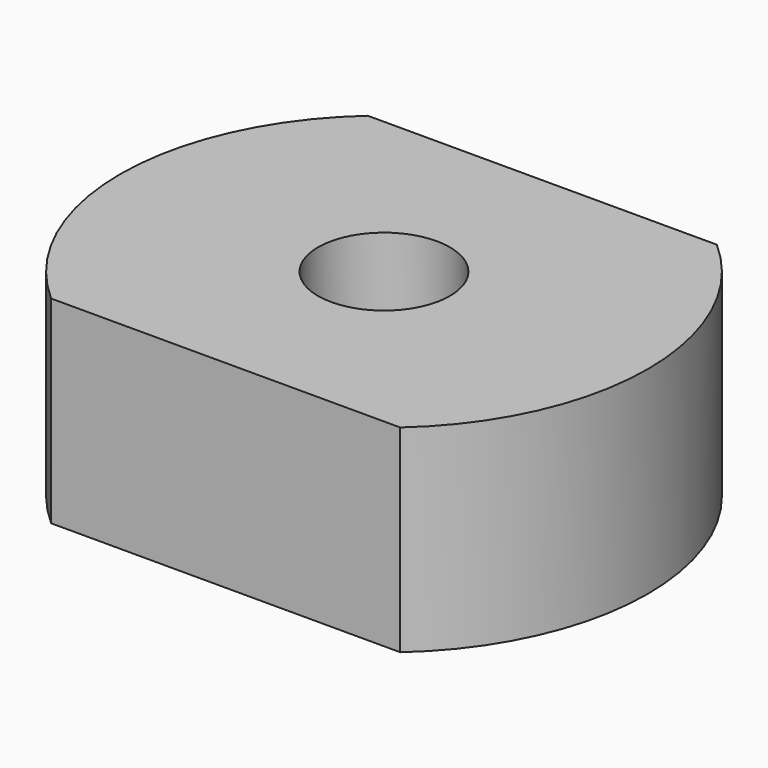
from build123d import *

# Parameters (mm, degrees)
F0_R     = 12.7
F1_DEPTH = 9.525
F3_D     = 6.35
F3_DEPTH = 5.08
F3_TIP   = 1.9077324654
F5_DEPTH = 25.4


# Not quite as in the source:
# - a feature names something its author has since deleted; it is built from what else it names


with BuildPart() as f1:
    # F0 (on Top) → F1 (new body)
    with BuildSketch(Plane.XY):
        Circle(F0_R)
    extrude(amount=F1_DEPTH)

    # F3
    with Locations(Plane.XY.offset(9.525)):
        with Locations((0, 0)):
            Hole(F3_D / 2, depth=F3_DEPTH)
            with Locations((0, 0, -(F3_DEPTH + F3_TIP / 2))):  # 118° drill point
                Cone(0, F3_D / 2, F3_TIP, mode=Mode.SUBTRACT)

    # F4 (on face) → F5 (cut)
    with BuildSketch(Plane.XY.offset(9.525)):
        with BuildLine():
            Line((19.05, -9.525), (19.05, 9.525))
            Line((19.05, 9.525), (8.4002604126, 9.525))
            ThreePointArc((8.4002604126, 9.525), (11.5752604126, 5.2252604126), (12.7, 0))
            ThreePointArc((12.7, 0), (11.5752604126, -5.2252604126), (8.4002604126, -9.525))
            Line((8.4002604126, -9.525), (19.05, -9.525))
        make_face()
        with BuildLine():
            ThreePointArc((-8.4002604126, -9.525), (-12.7, 0), (-8.4002604126, 9.525))
            Line((-8.4002604126, 9.525), (-19.05, 9.525))
            Line((-19.05, 9.525), (-19.05, -9.525))
            Line((-19.05, -9.525), (-8.4002604126, -9.525))
        make_face()
        with BuildLine():
            ThreePointArc((-8.4002604126, -9.525), (0, -12.7), (8.4002604126, -9.525))
            Line((8.4002604126, -9.525), (-8.4002604126, -9.525))
        make_face()
        with BuildLine():
            Line((-8.4002604126, 9.525), (8.4002604126, 9.525))
            ThreePointArc((8.4002604126, 9.525), (0, 12.7), (-8.4002604126, 9.525))
        make_face()
    extrude(amount=-F5_DEPTH, mode=Mode.SUBTRACT)


solid = f1.part
